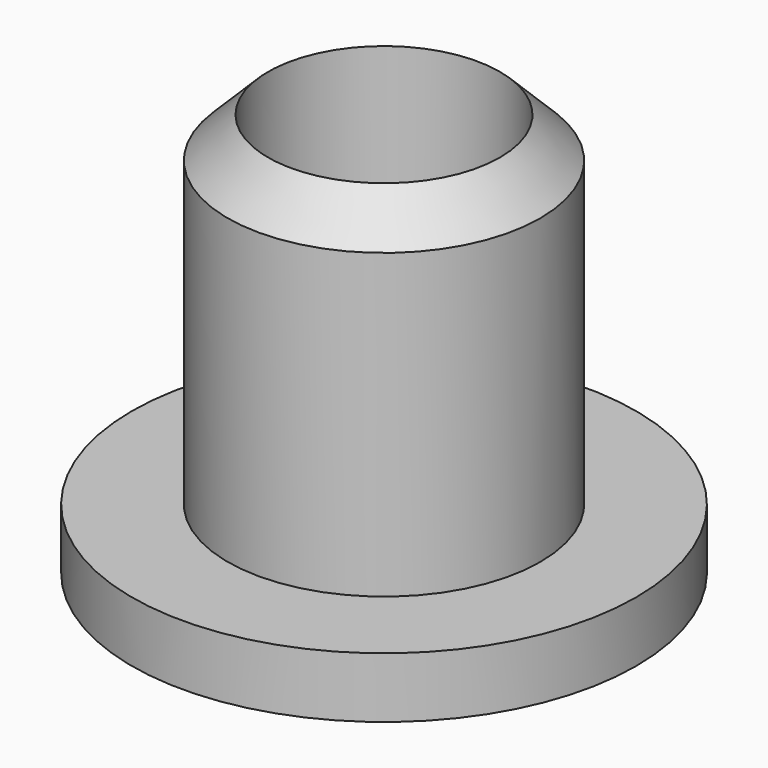
from build123d import *

# Parameters (mm, degrees)
F0_R     = 7.75
F0_R_2   = 5.75
F1_DEPTH = 20
F2_R     = 12.5
F2_R_2   = 7.75
F3_DEPTH = 3
F4_SIZE  = 1.99999


# Not quite as in the source:
# - a fillet or chamfer is up to 0.001 mm smaller than in the source, because OpenCascade refuses the exact size


with BuildPart() as f1:
    # F0 (on Top) → F1 (new body)
    with BuildSketch(Plane.XY):
        Circle(F0_R)
        Circle(F0_R_2, mode=Mode.SUBTRACT)
    extrude(amount=F1_DEPTH)

    # F2 (on Top) → F3 (join)
    with BuildSketch(Plane.XY):
        Circle(F2_R)
        Circle(F2_R_2, mode=Mode.SUBTRACT)
    extrude(amount=F3_DEPTH)

    # F4 (size 2 in the source; OpenCascade refuses exactly that, so slightly less here)
    f4_edges = [f1.edges().sort_by_distance(p)[0] for p in [
        (-7.75, 0, 20),
    ]]
    chamfer(f4_edges, length=F4_SIZE)


solid = f1.part
